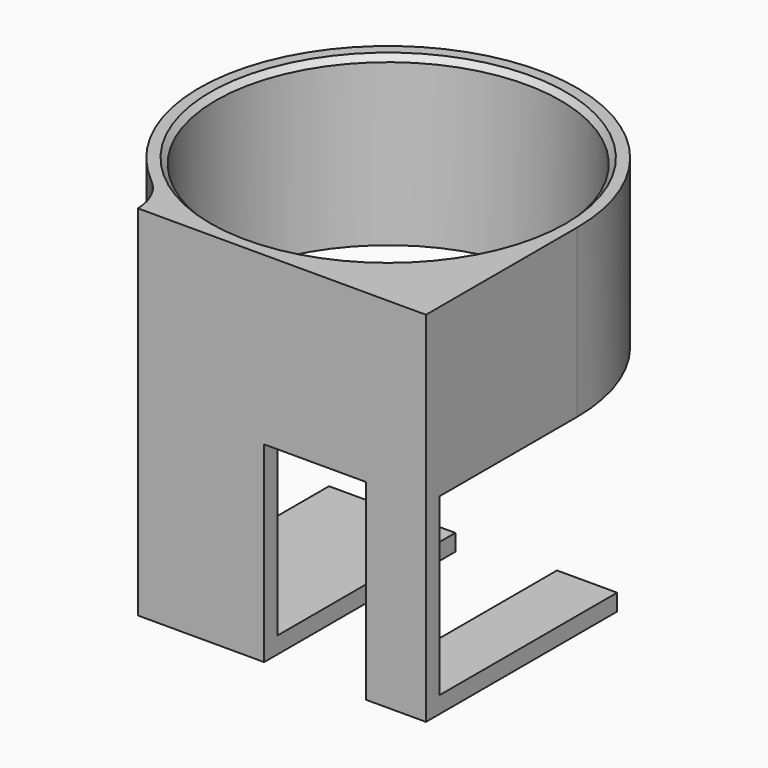
from build123d import *

# Parameters (mm, degrees)
F0_R        = 31
F1_DEPTH    = 3
F2_W        = 22.7279674787
F2_H        = 3
F2_W_2      = 10.8224550456
F3_DEPTH    = 34.5
F4_W        = 10.8224550456
F4_H        = 3
F5_DEPTH    = 40
F6_W        = 22.7279674787
F6_H        = 3
F7_DEPTH    = 40
F8_DEPTH    = 27
F9_T1_DEPTH = 30
F10_SIZE    = 1


# Not quite as in the source:
# - a fillet or chamfer that OpenCascade refuses, or shapes differently, is made with other operations: its cross-section is extruded or revolved along the edge and cut away or added


with BuildPart() as f1:
    # F0 (on Top) → F1 (new body)
    with BuildSketch(Plane.XY):
        with BuildLine():
            ThreePointArc((-34, 0), (-9.9583694397, 9.9583694397), (0, 34))
            ThreePointArc((0, 34), (-50.5693336344, 63.6893446023), (-51.8504225243, 5.0627849352))
            ThreePointArc((-51.8504225243, 5.0627849352), (-43.2772487246, 1.2901749301), (-34, 0))
        make_face()
        with Locations((-34, 34)):
            Circle(F0_R, mode=Mode.SUBTRACT)
        with BuildLine():
            ThreePointArc((-34, 0), (-43.2772487246, 1.2901749301), (-51.8504225243, 5.0627849352))
            Line((-51.8504225243, 5.0627849352), (-51.8504225243, 0))
            Line((-51.8504225243, 0), (-34, 0))
        make_face()
        with BuildLine():
            Line((0, 0), (0, 34))
            ThreePointArc((0, 34), (-9.9583694397, 9.9583694397), (-34, 0))
            Line((-34, 0), (0, 0))
        make_face()
    extrude(amount=F1_DEPTH)

    # F2 (on face) → F3 (join)
    with BuildSketch(Plane(origin=(0, 0, 0), x_dir=(1, 0, 0), z_dir=(0, 0, -1))):
        with Locations((-40.4864387849, -1.5)):
            Rectangle(F2_W, F2_H)
        with Locations((-5.4112275228, -1.5)):
            Rectangle(F2_W_2, F2_H)
    extrude(amount=F3_DEPTH)

    # F4 (on face) → F5 (join)
    with BuildSketch(Plane(origin=(0, 3, 0), x_dir=(-1, 0, 0), z_dir=(0, 1, 0))):
        with Locations((5.4112275228, -33)):
            Rectangle(F4_W, F4_H)
    extrude(amount=F5_DEPTH)

    # F6 (on face) → F7 (join)
    with BuildSketch(Plane(origin=(0, 3, 0), x_dir=(-1, 0, 0), z_dir=(0, 1, 0))):
        with Locations((40.4864387849, -33)):
            Rectangle(F6_W, F6_H)
    extrude(amount=F7_DEPTH)

    # F8 (add): a face of the model
    f8_faces = [f1.faces().sort_by_distance(p)[0] for p in [
        (-50.1006821075, 62.8496031264, 3),
    ]]
    extrude(f8_faces, amount=F8_DEPTH)

    # F9: fillet of radius 10.3311475389 on 1 edges, made by hand

    # F9_s2 → F9_t1 (join)
    with BuildSketch(Plane.XY):
        with BuildLine():
            ThreePointArc((-55.6121599632, 7.7528184042), (-52.8843757474, 4.2873402421), (-51.8504225243, 0))
            Line((-51.8504225243, 0), (-51.8504225243, 5.0627849352))
            ThreePointArc((-51.8504225243, 5.0627849352), (-53.7770807796, 6.3437696741), (-55.6121599632, 7.7528184042))
        make_face()
    extrude(amount=F9_T1_DEPTH)

    # F10
    f10_edges = [f1.edges().sort_by_distance(p)[0] for p in [
        (-65, 34, 30),
    ]]
    chamfer(f10_edges, length=F10_SIZE)


solid = f1.part
